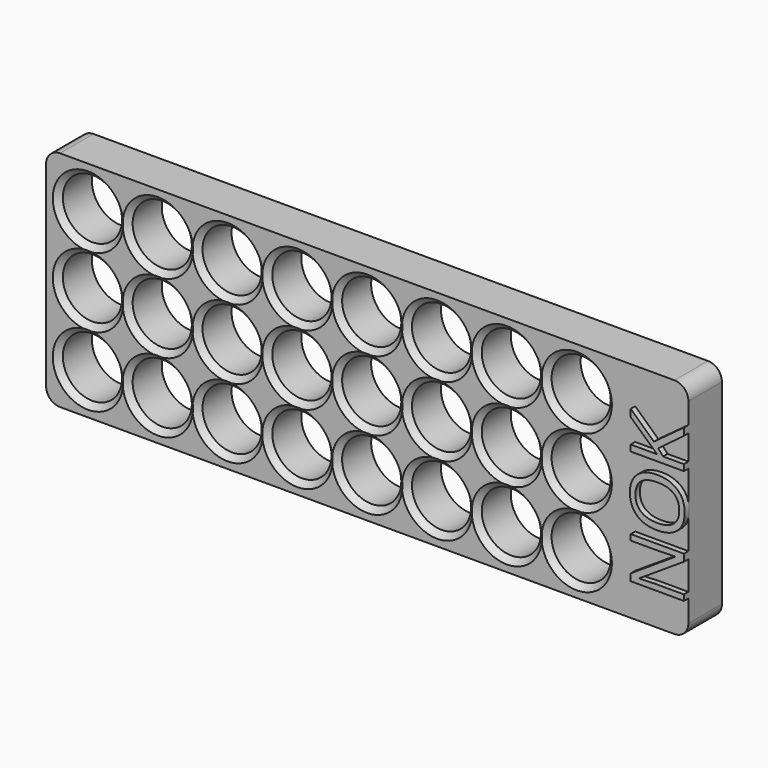
from build123d import *

# Parameters (mm, degrees)
F0_W         = 230
F0_H         = 80
F0_R         = 10.6
F1_DEPTH     = 15
F2_R         = 5
F4_TEXT_SIZE = 26.6793332606
F5_DEPTH     = 2


# Not quite as in the source:
# - a fillet or chamfer that OpenCascade refuses, or shapes differently, is made with other operations: its cross-section is extruded or revolved along the edge and cut away or added
# - a feature names something its author has since deleted; it is built from what else it names
# - Text() gives the source's letters only with a copy of the font that has no kerning and outlines rounded to 1/6400 em; it was checked with that copy


with BuildPart() as f1:
    # F0 (on Front) → F1 (new body)
    with BuildSketch(Plane.XZ):
        with Locations((10.2640186101, 115.6777501106)):
            Rectangle(F0_W, F0_H)
        with Locations((-89.7359813899, 90.6777501106)):
            Circle(F0_R, mode=Mode.SUBTRACT)
        with Locations((-64.7359813899, 90.6777501106)):
            Circle(F0_R, mode=Mode.SUBTRACT)
        with Locations((-39.7359813899, 90.6777501106)):
            Circle(F0_R, mode=Mode.SUBTRACT)
        with Locations((-14.7359813899, 90.6777501106)):
            Circle(F0_R, mode=Mode.SUBTRACT)
        with Locations((10.2640186101, 90.6777501106)):
            Circle(F0_R, mode=Mode.SUBTRACT)
        with Locations((-89.7359813899, 115.6777501106)):
            Circle(F0_R, mode=Mode.SUBTRACT)
        with Locations((-64.7359813899, 115.6777501106)):
            Circle(F0_R, mode=Mode.SUBTRACT)
        with Locations((-39.7359813899, 115.6777501106)):
            Circle(F0_R, mode=Mode.SUBTRACT)
        with Locations((-14.7359813899, 115.6777501106)):
            Circle(F0_R, mode=Mode.SUBTRACT)
        with Locations((10.2640186101, 115.6777501106)):
            Circle(F0_R, mode=Mode.SUBTRACT)
        with Locations((35.2640186101, 90.6777501106)):
            Circle(F0_R, mode=Mode.SUBTRACT)
        with Locations((60.2640186101, 90.6777501106)):
            Circle(F0_R, mode=Mode.SUBTRACT)
        with Locations((85.2640186101, 90.6777501106)):
            Circle(F0_R, mode=Mode.SUBTRACT)
        with Locations((35.2640186101, 115.6777501106)):
            Circle(F0_R, mode=Mode.SUBTRACT)
        with Locations((60.2640186101, 115.6777501106)):
            Circle(F0_R, mode=Mode.SUBTRACT)
        with Locations((85.2640186101, 115.6777501106)):
            Circle(F0_R, mode=Mode.SUBTRACT)
        with Locations((-89.7359813899, 140.6777501106)):
            Circle(F0_R, mode=Mode.SUBTRACT)
        with Locations((-64.7359813899, 140.6777501106)):
            Circle(F0_R, mode=Mode.SUBTRACT)
        with Locations((-39.7359813899, 140.6777501106)):
            Circle(F0_R, mode=Mode.SUBTRACT)
        with Locations((-14.7359813899, 140.6777501106)):
            Circle(F0_R, mode=Mode.SUBTRACT)
        with Locations((10.2640186101, 140.6777501106)):
            Circle(F0_R, mode=Mode.SUBTRACT)
        with Locations((35.2640186101, 140.6777501106)):
            Circle(F0_R, mode=Mode.SUBTRACT)
        with Locations((60.2640186101, 140.6777501106)):
            Circle(F0_R, mode=Mode.SUBTRACT)
        with Locations((85.2640186101, 140.6777501106)):
            Circle(F0_R, mode=Mode.SUBTRACT)
    extrude(amount=F1_DEPTH)

    # F2
    f2_edges = [f1.edges().sort_by_distance(p)[0] for p in [
        (125.264019, -7.5, 75.67775),
        (125.264019, -7.5, 155.67775),
        (-104.735981, -7.5, 155.67775),
        (-104.735981, -7.5, 75.67775),
    ]]
    fillet(f2_edges, radius=F2_R)

    # F3: chamfer of 2 on 24 edges, made by hand

    # F3_s1 → F3_t2 (revolve, cut)
    with BuildSketch(Plane.XY.offset(90.6777501106)):
        Polygon((-77.1359813899, -15), (-79.1359813899, -13), (-79.1359813899, -15), align=None)
    revolve(axis=Axis((-89.7359813899, -15, 90.6777501106), (0, -1, 0)), mode=Mode.SUBTRACT)

    # F3_s3 → F3_t4 (revolve, cut)
    with BuildSketch(Plane.XY.offset(115.6777501106)):
        Polygon((-77.1359813899, -15), (-79.1359813899, -13), (-79.1359813899, -15), align=None)
    revolve(axis=Axis((-89.7359813899, -15, 115.6777501106), (0, -1, 0)), mode=Mode.SUBTRACT)

    # F3_s5 → F3_t6 (revolve, cut)
    with BuildSketch(Plane.XY.offset(140.6777501106)):
        Polygon((-77.1359813899, -15), (-79.1359813899, -13), (-79.1359813899, -15), align=None)
    revolve(axis=Axis((-89.7359813899, -15, 140.6777501106), (0, -1, 0)), mode=Mode.SUBTRACT)

    # F3_s7 → F3_t8 (revolve, cut)
    with BuildSketch(Plane.XY.offset(140.6777501106)):
        Polygon((-52.1359813899, -15), (-54.1359813899, -13), (-54.1359813899, -15), align=None)
    revolve(axis=Axis((-64.7359813899, -15, 140.6777501106), (0, -1, 0)), mode=Mode.SUBTRACT)

    # F3_s9 → F3_t10 (revolve, cut)
    with BuildSketch(Plane.XY.offset(115.6777501106)):
        Polygon((-52.1359813899, -15), (-54.1359813899, -13), (-54.1359813899, -15), align=None)
    revolve(axis=Axis((-64.7359813899, -15, 115.6777501106), (0, -1, 0)), mode=Mode.SUBTRACT)

    # F3_s11 → F3_t12 (revolve, cut)
    with BuildSketch(Plane.XY.offset(90.6777501106)):
        Polygon((-52.1359813899, -15), (-54.1359813899, -13), (-54.1359813899, -15), align=None)
    revolve(axis=Axis((-64.7359813899, -15, 90.6777501106), (0, -1, 0)), mode=Mode.SUBTRACT)

    # F3_s13 → F3_t14 (revolve, cut)
    with BuildSketch(Plane.XY.offset(90.6777501106)):
        Polygon((-27.1359813899, -15), (-29.1359813899, -13), (-29.1359813899, -15), align=None)
    revolve(axis=Axis((-39.7359813899, -15, 90.6777501106), (0, -1, 0)), mode=Mode.SUBTRACT)

    # F3_s15 → F3_t16 (revolve, cut)
    with BuildSketch(Plane.XY.offset(115.6777501106)):
        Polygon((-27.1359813899, -15), (-29.1359813899, -13), (-29.1359813899, -15), align=None)
    revolve(axis=Axis((-39.7359813899, -15, 115.6777501106), (0, -1, 0)), mode=Mode.SUBTRACT)

    # F3_s17 → F3_t18 (revolve, cut)
    with BuildSketch(Plane.XY.offset(140.6777501106)):
        Polygon((-27.1359813899, -15), (-29.1359813899, -13), (-29.1359813899, -15), align=None)
    revolve(axis=Axis((-39.7359813899, -15, 140.6777501106), (0, -1, 0)), mode=Mode.SUBTRACT)

    # F3_s19 → F3_t20 (revolve, cut)
    with BuildSketch(Plane.XY.offset(140.6777501106)):
        Polygon((-2.1359813899, -15), (-4.1359813899, -13), (-4.1359813899, -15), align=None)
    revolve(axis=Axis((-14.7359813899, -15, 140.6777501106), (0, -1, 0)), mode=Mode.SUBTRACT)

    # F3_s21 → F3_t22 (revolve, cut)
    with BuildSketch(Plane.XY.offset(115.6777501106)):
        Polygon((-2.1359813899, -15), (-4.1359813899, -13), (-4.1359813899, -15), align=None)
    revolve(axis=Axis((-14.7359813899, -15, 115.6777501106), (0, -1, 0)), mode=Mode.SUBTRACT)

    # F3_s23 → F3_t24 (revolve, cut)
    with BuildSketch(Plane.XY.offset(90.6777501106)):
        Polygon((-2.1359813899, -15), (-4.1359813899, -13), (-4.1359813899, -15), align=None)
    revolve(axis=Axis((-14.7359813899, -15, 90.6777501106), (0, -1, 0)), mode=Mode.SUBTRACT)

    # F3_s25 → F3_t26 (revolve, cut)
    with BuildSketch(Plane.XY.offset(90.6777501106)):
        Polygon((22.8640186101, -15), (20.8640186101, -13), (20.8640186101, -15), align=None)
    revolve(axis=Axis((10.2640186101, -15, 90.6777501106), (0, -1, 0)), mode=Mode.SUBTRACT)

    # F3_s27 → F3_t28 (revolve, cut)
    with BuildSketch(Plane.XY.offset(115.6777501106)):
        Polygon((22.8640186101, -15), (20.8640186101, -13), (20.8640186101, -15), align=None)
    revolve(axis=Axis((10.2640186101, -15, 115.6777501106), (0, -1, 0)), mode=Mode.SUBTRACT)

    # F3_s29 → F3_t30 (revolve, cut)
    with BuildSketch(Plane.XY.offset(140.6777501106)):
        Polygon((22.8640186101, -15), (20.8640186101, -13), (20.8640186101, -15), align=None)
    revolve(axis=Axis((10.2640186101, -15, 140.6777501106), (0, -1, 0)), mode=Mode.SUBTRACT)

    # F3_s31 → F3_t32 (revolve, cut)
    with BuildSketch(Plane.XY.offset(140.6777501106)):
        Polygon((47.8640186101, -15), (45.8640186101, -13), (45.8640186101, -15), align=None)
    revolve(axis=Axis((35.2640186101, -15, 140.6777501106), (0, -1, 0)), mode=Mode.SUBTRACT)

    # F3_s33 → F3_t34 (revolve, cut)
    with BuildSketch(Plane.XY.offset(115.6777501106)):
        Polygon((47.8640186101, -15), (45.8640186101, -13), (45.8640186101, -15), align=None)
    revolve(axis=Axis((35.2640186101, -15, 115.6777501106), (0, -1, 0)), mode=Mode.SUBTRACT)

    # F3_s35 → F3_t36 (revolve, cut)
    with BuildSketch(Plane.XY.offset(140.6777501106)):
        Polygon((72.8640186101, -15), (70.8640186101, -13), (70.8640186101, -15), align=None)
    revolve(axis=Axis((60.2640186101, -15, 140.6777501106), (0, -1, 0)), mode=Mode.SUBTRACT)

    # F3_s37 → F3_t38 (revolve, cut)
    with BuildSketch(Plane.XY.offset(115.6777501106)):
        Polygon((72.8640186101, -15), (70.8640186101, -13), (70.8640186101, -15), align=None)
    revolve(axis=Axis((60.2640186101, -15, 115.6777501106), (0, -1, 0)), mode=Mode.SUBTRACT)

    # F3_s39 → F3_t40 (revolve, cut)
    with BuildSketch(Plane.XY.offset(140.6777501106)):
        Polygon((97.8640186101, -15), (95.8640186101, -13), (95.8640186101, -15), align=None)
    revolve(axis=Axis((85.2640186101, -15, 140.6777501106), (0, -1, 0)), mode=Mode.SUBTRACT)

    # F3_s41 → F3_t42 (revolve, cut)
    with BuildSketch(Plane.XY.offset(115.6777501106)):
        Polygon((97.8640186101, -15), (95.8640186101, -13), (95.8640186101, -15), align=None)
    revolve(axis=Axis((85.2640186101, -15, 115.6777501106), (0, -1, 0)), mode=Mode.SUBTRACT)

    # F3_s43 → F3_t44 (revolve, cut)
    with BuildSketch(Plane.XY.offset(90.6777501106)):
        Polygon((47.8640186101, -15), (45.8640186101, -13), (45.8640186101, -15), align=None)
    revolve(axis=Axis((35.2640186101, -15, 90.6777501106), (0, -1, 0)), mode=Mode.SUBTRACT)

    # F3_s45 → F3_t46 (revolve, cut)
    with BuildSketch(Plane.XY.offset(90.6777501106)):
        Polygon((72.8640186101, -15), (70.8640186101, -13), (70.8640186101, -15), align=None)
    revolve(axis=Axis((60.2640186101, -15, 90.6777501106), (0, -1, 0)), mode=Mode.SUBTRACT)

    # F3_s47 → F3_t48 (revolve, cut)
    with BuildSketch(Plane.XY.offset(90.6777501106)):
        Polygon((97.8640186101, -15), (95.8640186101, -13), (95.8640186101, -15), align=None)
    revolve(axis=Axis((85.2640186101, -15, 90.6777501106), (0, -1, 0)), mode=Mode.SUBTRACT)

    # F4 (on face) → F5 (join)
    with BuildSketch(Plane.XZ.offset(15)):
        with Locations(Location((125.2640186101, 85.9418623625), (0, 0, 90))):
            Text('NOK', F4_TEXT_SIZE, font='Open Sans', text_align=(TextAlign.LEFT, TextAlign.BOTTOM))
    extrude(amount=F5_DEPTH)


solid = f1.part
